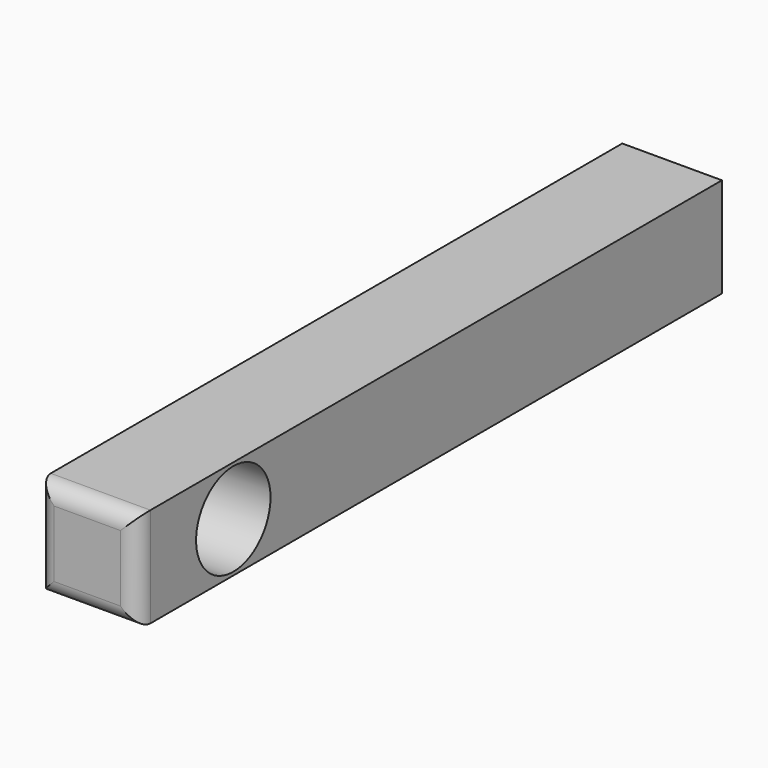
from build123d import *

# Parameters (mm, degrees)
F0_W     = 30
F0_H     = 30
F1_DEPTH = 220
F2_R     = 5
F3_R     = 14
F4_DEPTH = 40


with BuildPart() as f1:
    # F0 (on Front) → F1 (new body)
    with BuildSketch(Plane.XZ):
        Rectangle(F0_W, F0_H)
    extrude(amount=F1_DEPTH)

    # F2
    f2_edges = [f1.edges().sort_by_distance(p)[0] for p in [
        (15, -220, 0),
        (-15, -220, 0),
        (0, -220, 15),
        (0, -220, -15),
    ]]
    fillet(f2_edges, radius=F2_R)

    # F3 (on face) → F4 (cut)
    with BuildSketch(Plane.YZ.offset(15)):
        with Locations((-183.8199943304, 0)):
            Circle(F3_R)
    extrude(amount=-F4_DEPTH, mode=Mode.SUBTRACT)


solid = f1.part
